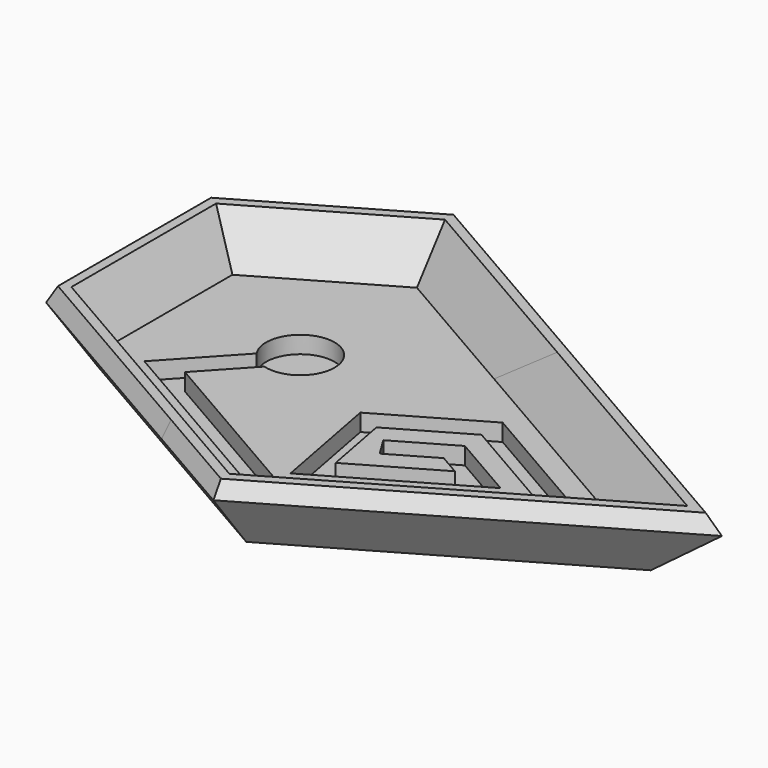
from build123d import *

# Parameters (mm, degrees)
F4_T     = -6.35
F5_R     = 9.525
F6_DEPTH = 4.7625
F8_DEPTH = 4.7625
F9_SIZE  = 5.08


with BuildPart() as f3:
    # F0 (on Top) → F3 section 0
    with BuildSketch(Plane.XY):
        Polygon((-38.494829, -22.225), (0, -44.45), (38.1, -66.447045), (115.089658, -21.997045), (38.494829, 22.225), (0, 44.45), (-38.494829, 22.225), align=None)
    # F2 (on offset) → F3 section 1
    with BuildSketch(Plane.XY.offset(19.05)):
        Polygon((-51.194829, 29.557348), (-51.194829, -29.557348), (14.459358, -67.462811), (38.1, -81.111742), (140.489658, -21.997045), (65.654187, 21.209234), (0, 59.114697), align=None)
    loft()

    # F4
    f4_openings = [f3.faces().sort_by_distance(p)[0] for p in [
        (27.801225, -12.100926, 19.05),
    ]]
    offset(amount=F4_T, openings=f4_openings)

    # F5 (on face) → F6 (cut)
    with BuildSketch(Plane.XY.offset(6.35)):
        Circle(F5_R)
    extrude(amount=-F6_DEPTH, mode=Mode.SUBTRACT)

    # F7 (on face) → F8 (cut, through all)
    with BuildSketch(Plane.XY.offset(6.35)):
        Polygon((84.102548, -21.997045), (34.827319, -50.446112), (-14.552667, -21.936564), (-2.703014, -9.133419), (-7.869169, -5.366731), (-24.614634, -23.459633), (34.827319, -57.77846), (96.802548, -21.997045), (54.167134, 2.618523), (27.091227, -13.013759), (33.104792, -44.8067), (73.067471, -21.734236), (54.622333, -11.084931), (39.102027, -20.045583), (42.431337, -25.455754), (54.622333, -18.417279), (60.367471, -21.734236), (37.68077, -34.832409), (34.167912, -16.260382), (54.167134, -4.713826), align=None)
    extrude(amount=-F8_DEPTH, mode=Mode.SUBTRACT)

    # F9
    f9_edges = [f3.edges().sort_by_distance(p)[0] for p in [
        (-18.367736, -48.51008, 19.05),
        (89.294829, -51.554394, 19.05),
        (103.071923, -0.393906, 19.05),
        (-25.597415, 44.336023, 19.05),
        (-51.194829, 0, 19.05),
    ]]
    chamfer(f9_edges, length=F9_SIZE)


solid = f3.part
